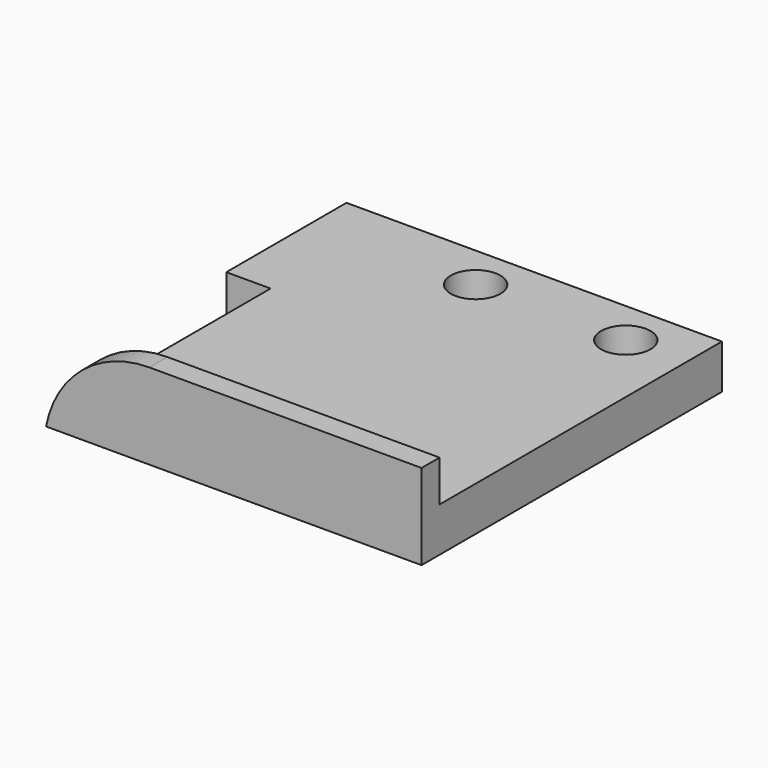
from build123d import *

# Parameters (mm, degrees)
F0_W        = 12.5
F0_H        = 25
F1_DEPTH    = 5.7
F2_W        = 23.5
F2_H        = 2.75
F3_DEPTH    = 25.001
F5_DEPTH    = 13.5
F6_T4_DEPTH = 35.8911325781
F7_R        = 1.65
F8_DEPTH    = 5.701


# Not quite as in the source:
# - a fillet or chamfer that OpenCascade refuses, or shapes differently, is made with other operations: its cross-section is extruded or revolved along the edge and cut away or added


with BuildPart() as f1:
    # F0 (on Top) → F1 (new body)
    with BuildSketch(Plane.XY):
        with Locations((-6.25, 12.5)):
            Rectangle(F0_W, F0_H)
        with Locations((6.25, 12.5)):
            Rectangle(F0_W, F0_H)
    extrude(amount=F1_DEPTH)

    # F2 (on face) → F3 (cut, through all)
    with BuildSketch(Plane.YZ.offset(12.5)):
        with Locations((13.25, 4.325)):
            Rectangle(F2_W, F2_H)
    extrude(amount=-F3_DEPTH, mode=Mode.SUBTRACT)

    # F4 (on face) → F5 (cut)
    with BuildSketch(Plane(origin=(0, 1.5, 0), x_dir=(-1, 0, 0), z_dir=(0, 1, 0))):
        Polygon((9.55, 2.95), (12.5, 0), (12.5, 2.95), align=None)
    extrude(amount=F5_DEPTH, mode=Mode.SUBTRACT)

    # F6: fillet of radius 7 on 1 edges, made by hand


with BuildPart() as f6_tool2:
    # F6_s3 → F6_t4 (new body)
    with BuildSketch(Plane.XZ.offset(-18.695566289)):
        with BuildLine():
            ThreePointArc((-12.5, 0), (-10.0883157712, 4.0898051913), (-5.6217734844, 5.7))
            Line((-5.6217734844, 5.7), (-12.5, 5.7))
            Line((-12.5, 5.7), (-12.5, 0))
        make_face()
    extrude(amount=F6_T4_DEPTH)

    split(bisect_by=Plane.XZ.offset(-15), keep=Keep.TOP)


with BuildPart() as f1_1:
    add(f1.part)

    # F6_t1: cut F6_tool2
    add(f6_tool2.part, mode=Mode.SUBTRACT)

    # F7 (on face) → F8 (cut, through all)
    with BuildSketch(Plane(origin=(0, 0, 0), x_dir=(1, 0, 0), z_dir=(0, 0, -1))):
        with Locations((-1.5, -22)):
            Circle(F7_R)
        with Locations((8.5, -22)):
            Circle(F7_R)
    extrude(amount=-F8_DEPTH, mode=Mode.SUBTRACT)


solid = f1_1.part
